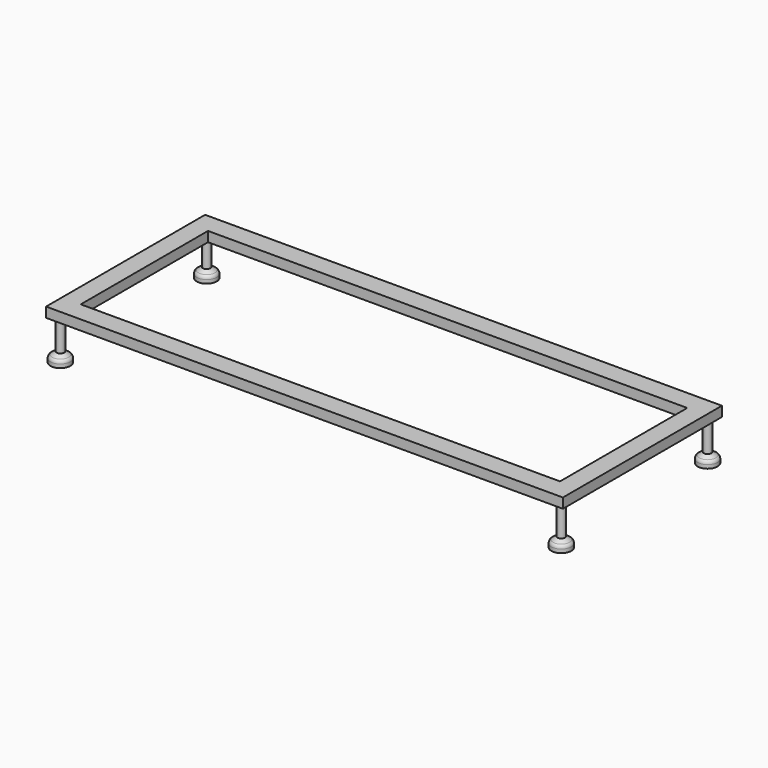
from build123d import *

# Parameters (mm, degrees)
F7_W     = 1300
F7_H     = 500
F7_W_2   = 1205.5341005325
F7_H_2   = 400
F8_DEPTH = 25


# Not quite as in the source:
# - a pattern or mirror of a feature is missing from the dataset's text; its kind, count and spacing are read off the source's solid


with BuildPart() as f6:
    # F5 (on line) → F6 (revolve)
    with BuildSketch(Plane(origin=(-630, 0, 0), x_dir=(0, -1, 0), z_dir=(-1, 0, 0))):
        with BuildLine():
            Line((230, 0), (220, 0))
            Line((220, 0), (220.3241423469, -7.5328363425))
            Line((220.3241423469, -7.5328363425), (220.3241423469, -75.4886860348))
            Line((220.3241423469, -75.4886860348), (209.5771272384, -82.4251501433))
            ThreePointArc((209.5771272384, -82.4251501433), (206.2185215477, -86.0431881155), (205, -90.8270815291))
            Line((205, -90.8270815291), (205, -100))
            Line((205, -100), (230, -100))
            Line((230, -100), (230, 0))
        make_face()
    revolve(axis=Axis((-630, -230, -56.9955855608), (0, 0, -1)))


with BuildPart() as f6_copies_1:
    # F6_copies: instance of F6
    add(f6.part.mirror(Plane(origin=(0, 0, 0), x_dir=(-0.3429399739, 0.9393573198, 0), z_dir=(0.9393573198, 0.3429399739, 0))))


with BuildPart() as f6_copies1_1:
    # F6_copies1: instance of F6
    add(f6.part.mirror(Plane(origin=(0, 0, 0), x_dir=(0, 0, 1), z_dir=(1, 0, 0))))


with BuildPart() as f6_copies2_1:
    # F6_copies2: instance of F6
    add(f6.part.mirror(Plane.ZX))


with BuildPart() as f8:
    # F7 (on face) → F8 (new body)
    with BuildSketch(Plane.XY):
        Rectangle(F7_W, F7_H)
        Rectangle(F7_W_2, F7_H_2, mode=Mode.SUBTRACT)
    extrude(amount=F8_DEPTH)


solid = Compound([f6.part, f6_copies_1.part, f6_copies1_1.part, f6_copies2_1.part, f8.part])
